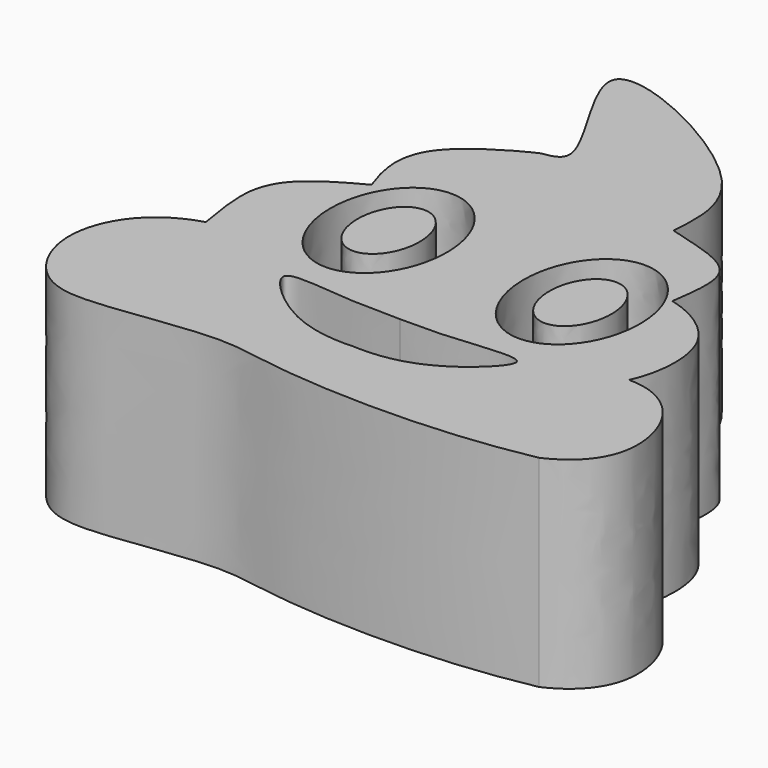
from build123d import *

# Parameters (mm, degrees)
F1_DEPTH = 25.4


# Not quite as in the source:
# - a feature names something its author has since deleted; it is built from what else it names


with BuildPart() as f1:
    # F0 (on Top) → F1 (new body)
    with BuildSketch(Plane.XY):
        with BuildLine():
            add(Edge.make_bspline(
                [(-12.7040585503, -6.7620049231), (-5.9350933235, -6.7620049231), (-9.3195759369, 1.6408482916), (-12.7040585503, 10.0437015062), (-16.0885411637, 1.6408482916), (-19.4730237771, -6.7620049231), (-12.7040585503, -6.7620049231)],
                knots=[0, 0, 0, 2.0943951024, 2.0943951024, 4.1887902048, 4.1887902048, 6.2831853072, 6.2831853072, 6.2831853072], degree=2, weights=[1, 0.5, 1, 0.5, 1, 0.5, 1]))
        make_face()
    extrude(amount=F1_DEPTH)


with BuildPart() as f1b:
    # F0 (on Top) → F1, piece 2 (new body)
    with BuildSketch(Plane.XY):
        with BuildLine():
            add(Edge.make_bspline(
                [(11.6227455437, -6.9933673367), (18.3917107705, -6.9933673367), (15.0072281571, 1.409485878), (11.6227455437, 9.8123390926), (8.2382629303, 1.409485878), (4.8537803169, -6.9933673367), (11.6227455437, -6.9933673367)],
                knots=[0, 0, 0, 2.0943951024, 2.0943951024, 4.1887902048, 4.1887902048, 6.2831853072, 6.2831853072, 6.2831853072], degree=2, weights=[1, 0.5, 1, 0.5, 1, 0.5, 1]))
        make_face()
    extrude(amount=F1_DEPTH)


with BuildPart() as f1c:
    # F0 (on Top) → F1, piece 3 (new body)
    with BuildSketch(Plane.XY):
        with BuildLine():
            add(Edge.make_bspline(
                [(9.178722043, 16.3179510783), (12.4271948484, 15.2755498145), (20.2967156839, 14.022973572), (18.7862815098, 7.1758211052), (18.4828080237, 4.5218956657)],
                knots=[0, 0, 0, 0, 0.5264260263, 1, 1, 1, 1], degree=3))
            add(Edge.make_bspline(
                [(-11.2985467915, 20.9806796509), (-10.057150046, 21.1740444447), (-5.8851955456, 21.8238843325), (-25.6351875023, 46.3924273574), (10.1706858503, 29.215430324), (9.4740668065, 20.1580135174), (9.178722043, 16.3179510783)],
                knots=[0, 0, 0, 0, 0.1217063112, 0.4090176605, 0.7494419068, 1, 1, 1, 1], degree=3))
            add(Edge.make_bspline(
                [(-20.0772415847, 5.3842621855), (-21.8382337034, 10.0368110982), (-21.422247354, 15.9537207711), (-12.3091086617, 20.5435363037), (-11.2985467915, 20.9806796509)],
                knots=[0, 0, 0, 0, 0.5126433129, 1, 1, 1, 1], degree=3))
            add(Edge.make_bspline(
                [(-27.8385281563, -11.0006788746), (-28.8563501799, -5.2754222973), (-28.7677518132, -1.1751763415), (-25.8164535696, 2.3950880339), (-20.0772415847, 5.3842621855)],
                knots=[0, 0, 0, 0, 0.4890841283, 1, 1, 1, 1], degree=3))
            add(Edge.make_bspline(
                [(29.0775820613, -29.7263264656), (16.6258025491, -32.1920238286), (-2.8263918493, -31.3268267458), (-10.7913914989, -29.0169685325), (-24.3625523476, -31.4019512541), (-32.8406534725, -31.3804329417), (-38.6972113755, -21.4661147228), (-33.8300936303, -12.7482184899), (-27.8385281563, -11.0006788746)],
                knots=[0, 0, 0, 0, 0.2608161586, 0.3933988062, 0.5600192096, 0.6897754866, 0.8288474437, 1, 1, 1, 1], degree=3))
            add(Edge.make_bspline(
                [(25.6281197071, -11.2470695749), (31.3780816561, -11.2470695749), (37.1892028294, -20.5940376025), (33.5515896494, -27.670699974), (29.0775820613, -29.7263264656)],
                knots=[0, 0, 0, 0, 0.5205802608, 1, 1, 1, 1], degree=3))
            add(Edge.make_bspline(
                [(18.4828080237, 4.5218956657), (21.2459100287, 3.8311192941), (27.8121902179, 0.1240076306), (26.9832648337, -8.4135830402), (25.6281197071, -11.2470695749)],
                knots=[0, 0, 0, 0, 0.4848063676, 1, 1, 1, 1], degree=3))
        make_face()
        with BuildLine():
            add(Edge.make_bspline(
                [(-12.5728802401, -11.1296701583), (0.2471999237, -10.9609851603), (-6.3596076235, 3.9090234082), (-12.9664151708, 18.7790319766), (-19.1796877873, 3.7403384102), (-25.3929604038, -11.2983551563), (-12.5728802401, -11.1296701583)],
                knots=[0, 0, 0, 2.0943951024, 2.0943951024, 4.1887902048, 4.1887902048, 6.2831853072, 6.2831853072, 6.2831853072], degree=2, weights=[1, 0.5, 1, 0.5, 1, 0.5, 1]))
        make_face(mode=Mode.SUBTRACT)
        with BuildLine():
            add(Edge.make_bspline(
                [(0, -15.2146350592), (-2.7093640529, -15.1272825897), (-6.4763540853, -15.2576190966), (-12.8391100977, -14.3530894957), (-15.9056872213, -15.1606946119), (-9.0218502029, -21.8425042061), (-3.136542703, -22.7859484552), (-1.917e-07, -22.6136597791)],
                knots=[0, 0, 0, 0, 0.2151521156, 0.4206744136, 0.5235423855, 0.7466305589, 0.9990126491, 0.9990126491, 0.9990126491, 0.9990126491], degree=3))
            add(Edge.make_bspline(
                [(0, -15.2146350592), (2.9838385526, -15.2277508751), (6.3519287872, -15.2120746239), (12.8536782629, -14.3584220078), (15.8990746005, -15.1582741368), (9.0246394492, -21.8435253707), (3.1365539853, -22.7859527427), (-1.917e-07, -22.6136597791)],
                knots=[0, 0, 0, 0, 0.2151521156, 0.4206744136, 0.5235423855, 0.7466305589, 0.9990126612, 0.9990126612, 0.9990126612, 0.9990126612], degree=3))
        make_face(mode=Mode.SUBTRACT)
        with BuildLine():
            add(Edge.make_bspline(
                [(11.753923854, -11.1296701583), (24.5740040177, -10.9609851603), (17.9671964705, 3.9090234082), (11.3603889232, 18.7790319766), (5.1471163067, 3.7403384102), (-1.0661563098, -11.2983551563), (11.753923854, -11.1296701583)],
                knots=[0, 0, 0, 2.0943951024, 2.0943951024, 4.1887902048, 4.1887902048, 6.2831853072, 6.2831853072, 6.2831853072], degree=2, weights=[1, 0.5, 1, 0.5, 1, 0.5, 1]))
        make_face(mode=Mode.SUBTRACT)
    extrude(amount=F1_DEPTH)


solid = Compound([f1.part, f1b.part, f1c.part])
